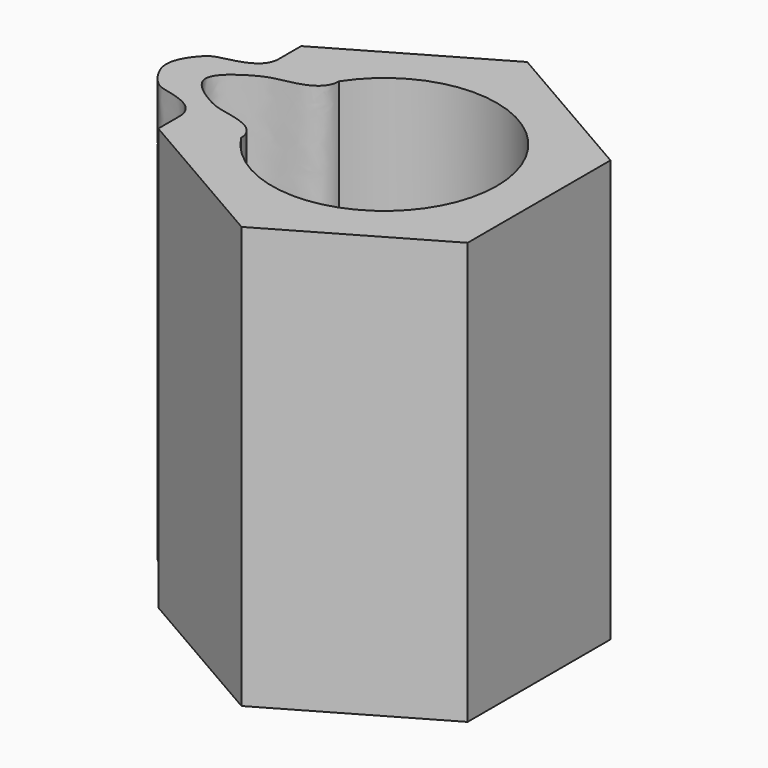
from build123d import *

# Parameters (mm, degrees)
F0_R       = 4
F1_DEPTH   = 15
F1_FACE1_R = 4
F3_DEPTH   = 15.001
F5_DEPTH   = 15


# Not quite as in the source:
# - a feature of the source that left no trace in its solid (it failed there, or was rolled back) is left out


with BuildPart() as f1:
    # F0 (on Top) → F1 (new body)
    with BuildSketch(Plane.XY):
        Polygon((5.5, -3.1754264805), (5.5, 3.1754264805), (0, 6.3508529611), (-5.5, 3.1754264805), (-5.5, -3.1754264805), (0, -6.3508529611), align=None)
        Circle(F0_R, mode=Mode.SUBTRACT)
    extrude(amount=F1_DEPTH)

    # F2 (on face) + F1_face1 (on face) → F3 (cut, through all)
    with BuildSketch(Plane.XY.offset(15)):
        with BuildLine():
            Line((-3.3567126222, 2.1754264805), (-5.5, 2.1754264805))
            Line((-5.5, 2.1754264805), (-5.5, -2.1754264805))
            Line((-5.5, -2.1754264805), (-3.3567126222, -2.1754264805))
            ThreePointArc((-3.3567126222, -2.1754264805), (-4, 0), (-3.3567126222, 2.1754264805))
        make_face()
    with BuildSketch(Plane(origin=(0, 0, 0), x_dir=(1, 0, 0), z_dir=(0, 0, -1))):
        Polygon((5.5, -3.1754264805), (5.5, 3.1754264805), (0, 6.3508529611), (-5.5, 3.1754264805), (-5.5, -3.1754264805), (0, -6.3508529611), align=None)
        Circle(F1_FACE1_R, mode=Mode.SUBTRACT)
    extrude(amount=-F3_DEPTH, dir=(0, 0, 1), mode=Mode.SUBTRACT)

    # F4 (on Top) → F5 (join, through all)
    with BuildSketch(Plane.XY):
        with BuildLine():
            add(Edge.make_bspline(
                [(-3.3567126222, 2.1754264805), (-3.3567126222, 1.5), (-4.7243783011, 1.2322496152), (-5.2691254391, 1.1014623302), (-6.9790180063, 0), (-5.2691254391, -1.1014623302), (-4.7243783011, -1.2322496152), (-3.3567126222, -1.5), (-3.3567126222, -2.1754264805)],
                knots=[0, 0, 0, 0, 0.1875096718, 0.3211964826, 0.5, 0.6788035174, 0.8124903282, 1, 1, 1, 1], degree=3))
            Line((-3.3567126222, 2.1754264805), (-5.5, 2.1754264805))
            add(Edge.make_bspline(
                [(-5.5, 2.1754264805), (-5.5, 1.5), (-6.8295402039, 1.2640494778), (-7.2493526274, 1.0792890587), (-8.0427649595, -0.000100502), (-7.2510852775, -1.0789459234), (-6.8212907124, -1.2661384452), (-5.5, -1.5), (-5.5, -2.2451365801)],
                knots=[0, 0, 0, 0, 0.2037356069, 0.3258802228, 0.4986187951, 0.6713573674, 0.7935019833, 1, 1, 1, 1], degree=3))
            Line((-5.5, -2.2451365801), (-3.3567126222, -2.1754264805))
        make_face()
    extrude(amount=F5_DEPTH)


solid = f1.part
